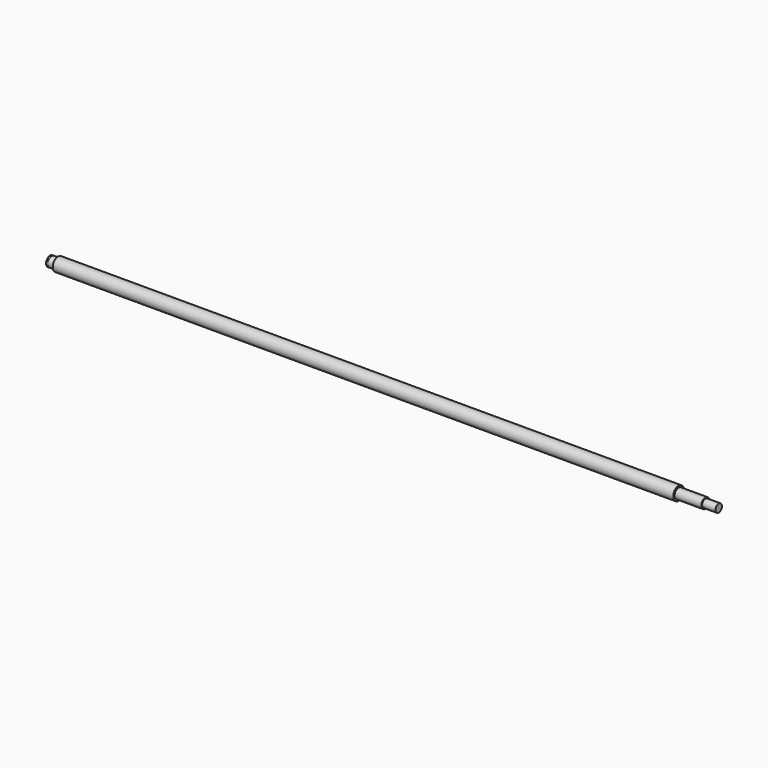
from build123d import *

# Parameters (mm, degrees)
F0_R     = 10
F1_DEPTH = 1000
F2_R     = 10
F2_R_2   = 6
F3_DEPTH = 20
F4_R     = 10
F4_R_2   = 7.5
F5_DEPTH = 40
F6_R     = 10
F6_R_2   = 7.5
F7_DEPTH = 12
F8_W     = 1.15
F8_H     = 0.35


with BuildPart() as f1:
    # F0 (on Right) → F1 (new body)
    with BuildSketch(Plane.YZ):
        Circle(F0_R)
    extrude(amount=-F1_DEPTH)

    # F2 (on face) → F3 (cut)
    with BuildSketch(Plane.YZ):
        Circle(F2_R)
        Circle(F2_R_2, mode=Mode.SUBTRACT)
    extrude(amount=-F3_DEPTH, mode=Mode.SUBTRACT)

    # F4 (on face) → F5 (cut)
    with BuildSketch(Plane.YZ.offset(-20)):
        Circle(F4_R)
        Circle(F4_R_2, mode=Mode.SUBTRACT)
    extrude(amount=-F5_DEPTH, mode=Mode.SUBTRACT)

    # F6 (on face) → F7 (cut)
    with BuildSketch(Plane(origin=(-1000, 0, 0), x_dir=(0, -1, 0), z_dir=(-1, 0, 0))):
        Circle(F6_R)
        Circle(F6_R_2, mode=Mode.SUBTRACT)
    extrude(amount=-F7_DEPTH, mode=Mode.SUBTRACT)

    # F8 (on Front) → F9 (revolve, cut)
    with BuildSketch(Plane.XZ):
        with Locations((-997.575, 7.325)):
            Rectangle(F8_W, F8_H)
    revolve(axis=Axis((-986.6362512112, 0, 0), (1, 0, 0)), mode=Mode.SUBTRACT)


solid = f1.part
